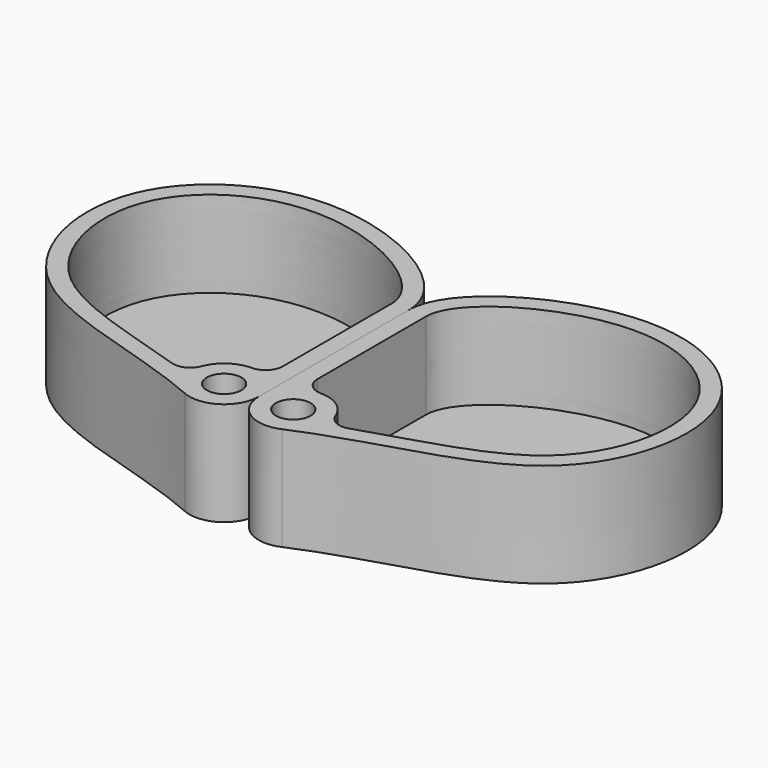
from build123d import *

# Parameters (mm, degrees)
F0_R     = 6.35
F1_DEPTH = 38.1
F2_DEPTH = 6.35


# Not quite as in the source:
# - the dataset's text gives a spline's control points without its knots; the knots are read off the source's solid


with BuildPart() as f1:
    # F0 (on Top) → F1 (new body)
    with BuildSketch(Plane.XY):
        with BuildLine():
            Line((0, 21.3322273978), (0, 90.2338773012))
            add(Edge.make_bspline(
                [(-17.7925559767, 9.6979730761), (-44.1249557649, 21.2242141409), (-101.9285953544, 27.8913395475), (-120.2849048364, 102.9335482434), (-57.9189683323, 141.6944403426), (0, 108.7021902204), (0, 90.2338773012)],
                knots=[0.0564270684, 0.0564270684, 0.0564270684, 0.0564270684, 0.2970876978, 0.5268230764, 0.7575195077, 1, 1, 1, 1], degree=3))
            ThreePointArc((-17.7925559767, 9.6979730761), (-5.7496568755, 10.7028939073), (0, 21.3322273978))
        make_face()
        with Locations((-12.7, 21.3322273978)):
            Circle(F0_R, mode=Mode.SUBTRACT)
        with BuildLine():
            add(Edge.make_bspline(
                [(-32.5238150415, 22.0449938542), (-34.6379317553, 22.748582145), (-40.308470557, 24.5698797188), (-49.3577928373, 27.323362061), (-59.3563808747, 30.458818188), (-68.6566721588, 33.7783884666), (-75.6401846906, 36.8732526986), (-80.6663591319, 39.633151423), (-83.5576182986, 41.4915374695), (-85.7146243872, 43.0688259393), (-87.2511410861, 44.2977880081), (-88.7154162125, 45.583896512), (-90.586225543, 47.3840218133), (-92.7635117395, 49.780798698), (-95.8987942041, 53.8975261415), (-99.1467856582, 59.5050198493), (-101.9147923444, 66.7410779055), (-103.5045913746, 74.2319443381), (-103.8209927993, 80.4681000106), (-103.4642007144, 85.3229329841), (-102.892792234, 88.8659432305), (-102.1650703109, 91.7119413387), (-101.4333264814, 93.9116049064), (-100.6023362942, 96.0550446002), (-99.3697377358, 98.6513901165), (-97.0014232071, 102.6110166748), (-93.3243120992, 107.17000512), (-87.8593225928, 111.9046291425), (-81.4483572734, 115.7782119632), (-74.2081320587, 118.662968178), (-67.5846494554, 120.1379677001), (-61.992096805, 120.6980354444), (-57.665733733, 120.7931146888), (-53.2212134118, 120.544694496), (-48.6464636132, 119.9485798425), (-44.0183173177, 119.0240270871), (-37.8584795046, 117.378727405), (-30.3406641042, 114.6036449742), (-22.1106226076, 110.3301856456), (-16.3246751133, 106.1927135418), (-12.5757553726, 102.7050588146), (-10.2549075727, 100.0552746686), (-8.4640703283, 97.4321950222), (-7.2192514586, 94.8988243587), (-6.5036966691, 92.5005712263), (-6.35, 90.9855396487), (-6.35, 90.2338773012)],
                knots=[0.106545855, 0.106545855, 0.106545855, 0.106545855, 0.125, 0.15625, 0.1875, 0.21875, 0.25, 0.265625, 0.28125, 0.2890625, 0.296875, 0.3046875, 0.3125, 0.328125, 0.34375, 0.375, 0.40625, 0.4375, 0.46875, 0.484375, 0.5, 0.515625, 0.5234375, 0.53125, 0.546875, 0.5625, 0.59375, 0.625, 0.65625, 0.6875, 0.71875, 0.734375, 0.75, 0.765625, 0.78125, 0.796875, 0.8125, 0.84375, 0.875, 0.90625, 0.921875, 0.9375, 0.953125, 0.96875, 0.984375, 1, 1, 1, 1], degree=3))
            Line((-6.35, 90.2338773012), (-6.35, 40.3822273978))
            ThreePointArc((-6.35, 40.3822273978), (-8.2098719395, 35.8920993373), (-12.7, 34.0322273978))
            ThreePointArc((-12.7, 34.0322273978), (-19.9195147201, 31.7806056072), (-24.5790898085, 25.8241340445))
            ThreePointArc((-24.5790898085, 25.8241340445), (-27.7909468094, 22.3357854311), (-32.5238150415, 22.0449938542))
        make_face(mode=Mode.SUBTRACT)
    extrude(amount=F1_DEPTH)

    # F0 (on Top) → F2 (join)
    with BuildSketch(Plane.XY):
        with BuildLine():
            Line((-6.35, 40.3822273978), (-6.35, 90.2338773012))
            add(Edge.make_bspline(
                [(-32.5238150415, 22.0449938542), (-34.6379317553, 22.748582145), (-40.308470557, 24.5698797188), (-49.3577928373, 27.323362061), (-59.3563808747, 30.458818188), (-68.6566721588, 33.7783884666), (-75.6401846906, 36.8732526986), (-80.6663591319, 39.633151423), (-83.5576182986, 41.4915374695), (-85.7146243872, 43.0688259393), (-87.2511410861, 44.2977880081), (-88.7154162125, 45.583896512), (-90.586225543, 47.3840218133), (-92.7635117395, 49.780798698), (-95.8987942041, 53.8975261415), (-99.1467856582, 59.5050198493), (-101.9147923444, 66.7410779055), (-103.5045913746, 74.2319443381), (-103.8209927993, 80.4681000106), (-103.4642007144, 85.3229329841), (-102.892792234, 88.8659432305), (-102.1650703109, 91.7119413387), (-101.4333264814, 93.9116049064), (-100.6023362942, 96.0550446002), (-99.3697377358, 98.6513901165), (-97.0014232071, 102.6110166748), (-93.3243120992, 107.17000512), (-87.8593225928, 111.9046291425), (-81.4483572734, 115.7782119632), (-74.2081320587, 118.662968178), (-67.5846494554, 120.1379677001), (-61.992096805, 120.6980354444), (-57.665733733, 120.7931146888), (-53.2212134118, 120.544694496), (-48.6464636132, 119.9485798425), (-44.0183173177, 119.0240270871), (-37.8584795046, 117.378727405), (-30.3406641042, 114.6036449742), (-22.1106226076, 110.3301856456), (-16.3246751133, 106.1927135418), (-12.5757553726, 102.7050588146), (-10.2549075727, 100.0552746686), (-8.4640703283, 97.4321950222), (-7.2192514586, 94.8988243587), (-6.5036966691, 92.5005712263), (-6.35, 90.9855396487), (-6.35, 90.2338773012)],
                knots=[0.106545855, 0.106545855, 0.106545855, 0.106545855, 0.125, 0.15625, 0.1875, 0.21875, 0.25, 0.265625, 0.28125, 0.2890625, 0.296875, 0.3046875, 0.3125, 0.328125, 0.34375, 0.375, 0.40625, 0.4375, 0.46875, 0.484375, 0.5, 0.515625, 0.5234375, 0.53125, 0.546875, 0.5625, 0.59375, 0.625, 0.65625, 0.6875, 0.71875, 0.734375, 0.75, 0.765625, 0.78125, 0.796875, 0.8125, 0.84375, 0.875, 0.90625, 0.921875, 0.9375, 0.953125, 0.96875, 0.984375, 1, 1, 1, 1], degree=3))
            ThreePointArc((-32.5238150415, 22.0449938542), (-27.7909468094, 22.3357854311), (-24.5790898085, 25.8241340445))
            ThreePointArc((-24.5790898085, 25.8241340445), (-19.9195147201, 31.7806056072), (-12.7, 34.0322273978))
            ThreePointArc((-12.7, 34.0322273978), (-8.2098719395, 35.8920993373), (-6.35, 40.3822273978))
        make_face()
    extrude(amount=F2_DEPTH)


with BuildPart() as f3_1:
    # F3: instance of F1
    add(f1.part.mirror(Plane.YZ))


solid = Compound([f1.part, f3_1.part])
